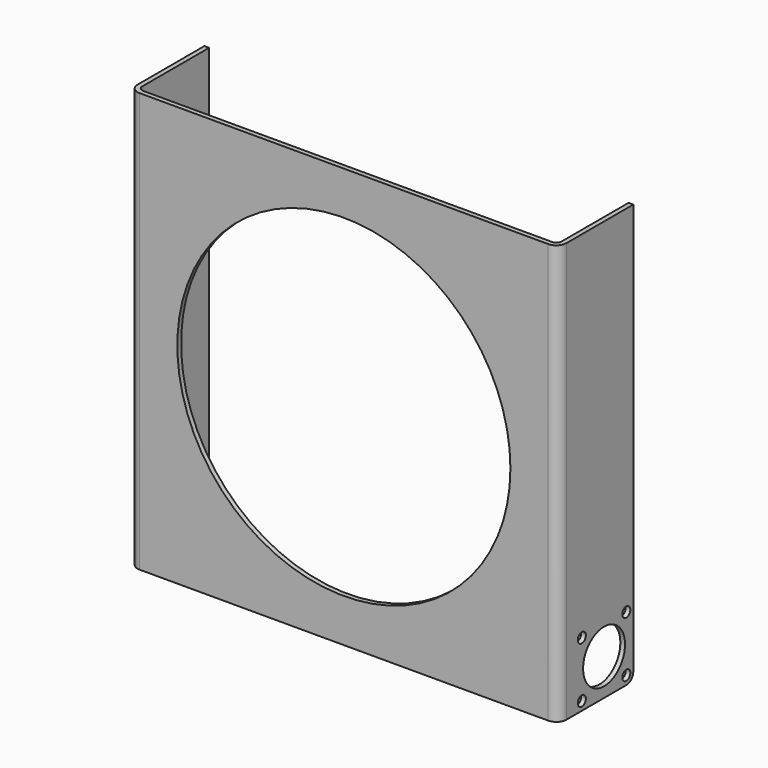
from build123d import *

# Parameters (mm, degrees)
F1_DEPTH = 152.4
F2_R     = 1.98374
F3_R     = 3.69316
F4_R     = 3.175
F5_R     = 9.525
F5_R_2   = 1.8288
F6_DEPTH = 155.81884
F7_R     = 60.500006
F8_DEPTH = 1.70942


with BuildPart() as f1:
    # F0 (on Top) → F1 (new body)
    with BuildSketch(Plane.XY):
        Polygon((0, 32.3337428), (0, 0), (-152.4, 0), (-152.4, 32.3337428), (-154.10942, 32.3337428), (-154.10942, -1.70942), (1.70942, -1.70942), (1.70942, 32.3337428), align=None)
    extrude(amount=F1_DEPTH)

    # F2
    f2_edges = [f1.edges().sort_by_distance(p)[0] for p in [
        (0, 0, 76.2),
        (-152.4, 0, 76.2),
    ]]
    fillet(f2_edges, radius=F2_R)

    # F3
    f3_edges = [f1.edges().sort_by_distance(p)[0] for p in [
        (1.70942, -1.70942, 76.2),
        (-154.10942, -1.70942, 76.2),
    ]]
    fillet(f3_edges, radius=F3_R)

    # F4
    f4_edges = [f1.edges().sort_by_distance(p)[0] for p in [
        (-153.25471, 32.333743, 0),
        (0.85471, 32.333743, 0),
    ]]
    fillet(f4_edges, radius=F4_R)

    # F5 (on face) → F6 (cut, through all)
    with BuildSketch(Plane.YZ.offset(1.70942)):
        with Locations((19.0559546638, 13.2777881362)):
            Circle(F5_R)
        with Locations((29.1587428, 23.3805762724)):
            Circle(F5_R_2)
        with Locations((29.1587428, 3.175)):
            Circle(F5_R_2)
        with Locations((8.9531665276, 3.175)):
            Circle(F5_R_2)
        with Locations((8.9531665276, 23.3805762724)):
            Circle(F5_R_2)
    extrude(amount=-F6_DEPTH, mode=Mode.SUBTRACT)

    # F7 (on face) → F8 (cut, through all)
    with BuildSketch(Plane.XZ.offset(1.70942)):
        with Locations((-76.2, 76.2)):
            Circle(F7_R)
    extrude(amount=-F8_DEPTH, mode=Mode.SUBTRACT)


solid = f1.part
